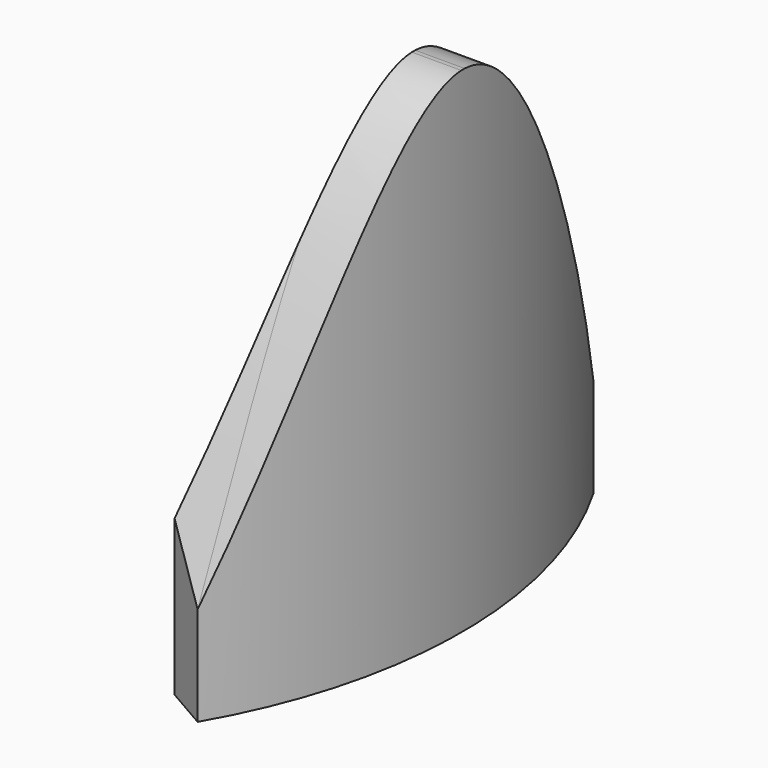
from build123d import *

# Parameters (mm, degrees)
F1_DEPTH = 12.7
F3_DEPTH = 6.35


# Not quite as in the source:
# - a feature names something its author has since deleted; it is built from what else it names


with BuildPart() as f1:
    # F0 (on Top) → F1 (new body)
    with BuildSketch(Plane.XY):
        with BuildLine():
            Line((-1.099852253, -12.0650000057), (0, -12.7))
            ThreePointArc((0, -12.7), (1.7014773719, -6.35), (0, 0))
            Line((0, 0), (-1.099852253, -0.6349999943))
            ThreePointArc((-1.099852253, -0.6349999943), (0.4314773832, -6.35), (-1.099852253, -12.0650000057))
        make_face()
    extrude(amount=F1_DEPTH)

    # F2 (on Right) → F3 (cut, symmetric)
    with BuildSketch(Plane.YZ):
        with BuildLine():
            Line((0, 12.7), (-6.259501017, 12.7))
            add(Edge.make_bspline(
                [(0, 2.54), (-2.0835692993, 7.5354677351), (-4.1744975267, 12.6135905998), (-6.259501017, 12.7)],
                knots=[0, 0, 0, 0, 0.4917268941, 0.4917268941, 0.4917268941, 0.4917268941], degree=3))
            Line((0, 2.54), (0, 12.7))
        make_face()
        with BuildLine():
            add(Edge.make_bspline(
                [(-6.259501017, 12.7), (-6.2953843519, 12.7014871234), (-6.331265932, 12.7014957456), (-6.3671456895, 12.7)],
                knots=[0.4917268941, 0.4917268941, 0.4917268941, 0.4917268941, 0.5001896141, 0.5001896141, 0.5001896141, 0.5001896141], degree=3))
            Line((-6.3671456895, 12.7), (-6.259501017, 12.7))
        make_face()
        with BuildLine():
            add(Edge.make_bspline(
                [(-6.3671456895, 12.7), (-8.4862132407, 12.6116608867), (-10.5989234677, 7.2759161441), (-12.7, 2.54)],
                knots=[0.5001896141, 0.5001896141, 0.5001896141, 0.5001896141, 1, 1, 1, 1], degree=3))
            Line((-6.3671456895, 12.7), (-12.7, 12.7))
            Line((-12.7, 12.7), (-12.7, 2.54))
        make_face()
    extrude(amount=F3_DEPTH, both=True, mode=Mode.SUBTRACT)


solid = f1.part
